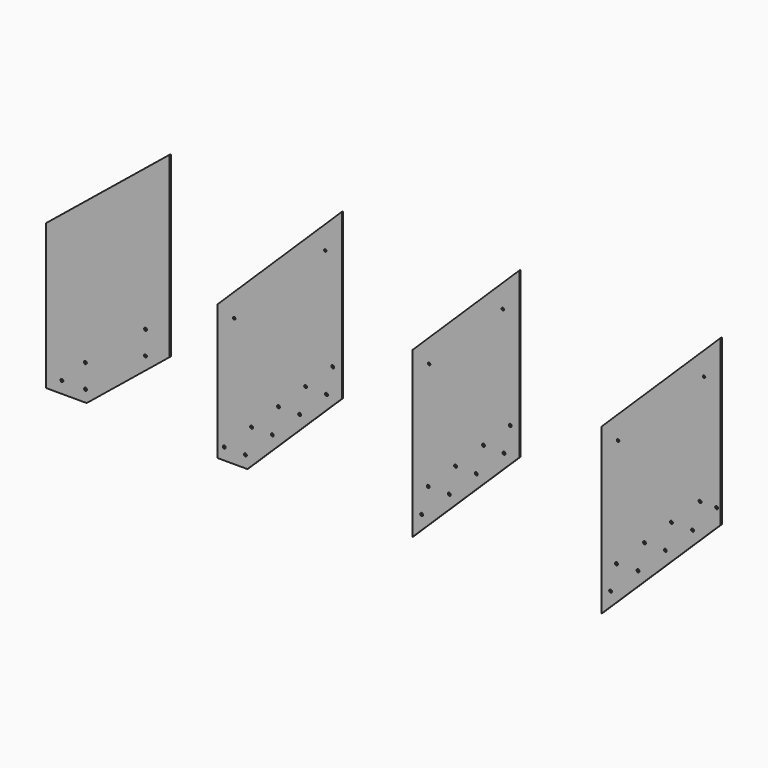
from build123d import *

# Parameters (mm, degrees)
F0_R     = 11.1125
F1_DEPTH = 12.7
F2_R     = 3.175
F3_R     = 11.1125
F3_R_2   = 9.525
F4_DEPTH = 12.7
F5_R     = 11.1125
F5_R_2   = 9.525
F6_DEPTH = 12.7
F7_R     = 11.1125
F7_R_2   = 9.525
F8_DEPTH = 12.7


# Not quite as in the source:
# - ends of sketch curves that miss each other by under 0.0002 mm in the source are joined


with BuildPart() as f1:
    # F0 (on Front) → F1 (new body)
    with BuildSketch(Plane.XZ):
        Polygon((-161.925, -941.1480288), (473.075, -425.2105288), (473.075, 941.1480288), (-473.075, 172.4011538), (-473.075, -941.1480288), align=None)
        with Locations((-352.0627452, -850.7056392)):
            Circle(F0_R, mode=Mode.SUBTRACT)
        with Locations((-171.45, -850.7056392)):
            Circle(F0_R, mode=Mode.SUBTRACT)
        with Locations((-171.45, -670.706304)):
            Circle(F0_R, mode=Mode.SUBTRACT)
        with Locations((288.925, -476.650939)):
            Circle(F0_R, mode=Mode.SUBTRACT)
        with Locations((288.925, -296.6516038)):
            Circle(F0_R, mode=Mode.SUBTRACT)
    extrude(amount=F1_DEPTH)

    # F2
    f2_edges = [f1.edges().sort_by_distance(p)[0] for p in [
        (473.075, -6.35, 941.148029),
        (-473.075, -6.35, 172.401154),
        (-473.075, -6.35, -941.148029),
        (-161.925, -6.35, -941.148029),
        (473.075, -6.35, -425.210529),
    ]]
    fillet(f2_edges, radius=F2_R)


with BuildPart() as f4:
    # F3 (on Front) → F4 (new body)
    with BuildSketch(Plane.XZ):
        Polygon((1070.6100212097, -986.0075712204), (1661.1600212097, -407.2318174204), (1794.5100212097, -276.5405116204), (1794.5100212097, 986.0076109796), (842.0100212097, 52.4983019796), (842.0100212097, -986.0075712204), align=None)
        with Locations((892.8100212097, -894.8718632204)):
            Circle(F3_R, mode=Mode.SUBTRACT)
        with Locations((1054.7350212097, -894.8718632204)):
            Circle(F3_R, mode=Mode.SUBTRACT)
        with Locations((1102.3489722097, -692.6115108204)):
            Circle(F3_R, mode=Mode.SUBTRACT)
        with Locations((1261.1100212097, -692.6115108204)):
            Circle(F3_R, mode=Mode.SUBTRACT)
        with Locations((969.0100212097, -0.8574714204)):
            Circle(F3_R_2, mode=Mode.SUBTRACT)
        with Locations((1308.7350212097, -487.0838802204)):
            Circle(F3_R, mode=Mode.SUBTRACT)
        with Locations((1470.8187712097, -487.0838802204)):
            Circle(F3_R, mode=Mode.SUBTRACT)
        with Locations((1516.7392534097, -283.3715622204)):
            Circle(F3_R, mode=Mode.SUBTRACT)
        with Locations((1677.0350212097, -284.9791028204)):
            Circle(F3_R, mode=Mode.SUBTRACT)
        with Locations((1724.6600212097, -82.7079300204)):
            Circle(F3_R, mode=Mode.SUBTRACT)
        with Locations((1667.5100212097, 683.7160133796)):
            Circle(F3_R_2, mode=Mode.SUBTRACT)
    extrude(amount=F4_DEPTH)


with BuildPart() as f6:
    # F5 (on Front) → F6 (new body)
    with BuildSketch(Plane.XZ):
        Polygon((2336.1649513245, -1032.6830148697), (3155.3149513245, -229.8650116697), (3155.3149513245, 1032.6831109303), (2336.1649513245, 229.8651077303), align=None)
        with Locations((2406.0149513245, -857.5314474697)):
            Circle(F5_R, mode=Mode.SUBTRACT)
        with Locations((2456.8038769245, -652.1594172697)):
            Circle(F5_R, mode=Mode.SUBTRACT)
        with Locations((2618.7399513245, -652.1594172697)):
            Circle(F5_R, mode=Mode.SUBTRACT)
        with Locations((2666.3649513245, -446.7765158697)):
            Circle(F5_R, mode=Mode.SUBTRACT)
        with Locations((2825.1149513245, -446.7873616697)):
            Circle(F5_R, mode=Mode.SUBTRACT)
        with Locations((2880.8362013245, -236.5813558697)):
            Circle(F5_R, mode=Mode.SUBTRACT)
        with Locations((3037.6382499245, -238.5012656697)):
            Circle(F5_R, mode=Mode.SUBTRACT)
        with Locations((3085.4649513245, -36.0324300697)):
            Circle(F5_R, mode=Mode.SUBTRACT)
        with Locations((2463.1649513245, 176.5093343303)):
            Circle(F5_R_2, mode=Mode.SUBTRACT)
        with Locations((3028.3149513245, 730.3915133303)):
            Circle(F5_R_2, mode=Mode.SUBTRACT)
    extrude(amount=F6_DEPTH)


with BuildPart() as f8:
    # F7 (on Front) → F8 (new body)
    with BuildSketch(Plane.XZ):
        Polygon((3785.1948738098, -1078.7762403488), (4698.4066110098, -183.7718581488), (4698.4066110098, 1078.7762390512), (3785.1948738098, 183.7718822512), align=None)
        with Locations((3855.0448738098, -903.6246729488)):
            Circle(F7_R, mode=Mode.SUBTRACT)
        with Locations((3899.4948738098, -704.4652033488)):
            Circle(F7_R, mode=Mode.SUBTRACT)
        with Locations((4064.5948738098, -698.2526173488)):
            Circle(F7_R, mode=Mode.SUBTRACT)
        with Locations((4115.3948738098, -492.8697413488)):
            Circle(F7_R, mode=Mode.SUBTRACT)
        with Locations((4274.1448738098, -492.8805871488)):
            Circle(F7_R, mode=Mode.SUBTRACT)
        with Locations((4321.7698738098, -288.1574761488)):
            Circle(F7_R, mode=Mode.SUBTRACT)
        with Locations((4483.0327212098, -288.1574761488)):
            Circle(F7_R, mode=Mode.SUBTRACT)
        with Locations((4540.8448738098, -75.9022491488)):
            Circle(F7_R, mode=Mode.SUBTRACT)
        with Locations((4667.8448738098, -75.9022491488)):
            Circle(F7_R, mode=Mode.SUBTRACT)
        with Locations((3912.1948738098, 130.4161088512)):
            Circle(F7_R_2, mode=Mode.SUBTRACT)
        with Locations((4571.4066110098, 776.4846668512)):
            Circle(F7_R_2, mode=Mode.SUBTRACT)
    extrude(amount=F8_DEPTH)


solid = Compound([f1.part, f4.part, f6.part, f8.part])
